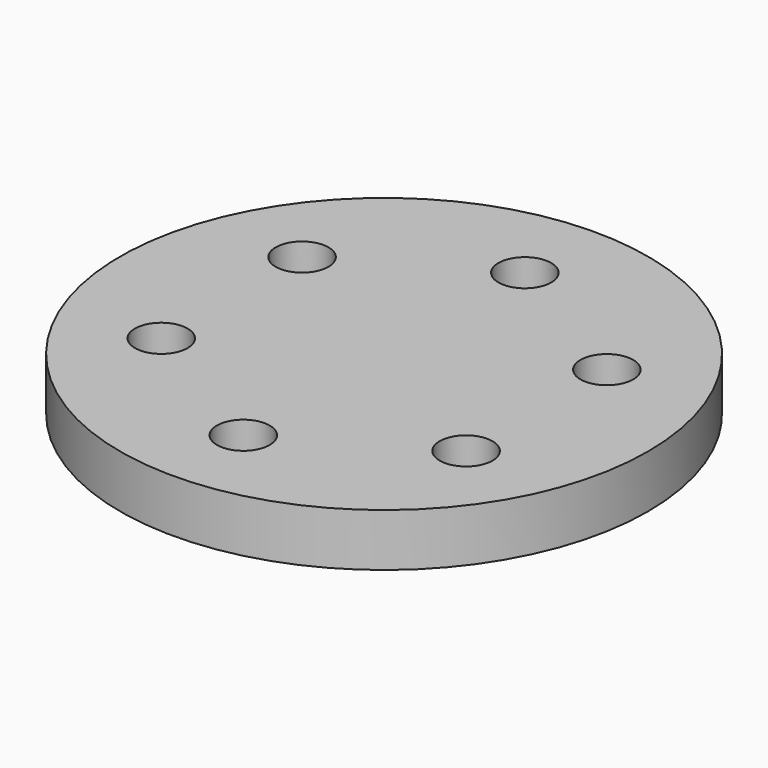
from build123d import *

# Parameters (mm, degrees)
F0_R            = 60
F1_DEPTH        = 12
F2_R            = 6
F3_DEPTH        = 12.001
F3_COPIES_COUNT = 6


# Not quite as in the source:
# - a pattern or mirror of a feature is missing from the dataset's text; its kind, count and spacing are read off the source's solid


with BuildPart() as f1:
    # F0 (on Top) → F1 (new body)
    with BuildSketch(Plane.XY):
        Circle(F0_R)
    extrude(amount=F1_DEPTH)

    # F2 (on face) → F3 (cut, through all)
    with BuildSketch(Plane.XY.offset(12)):
        with Locations((0, 40)):
            Circle(F2_R)
    f3 = extrude(amount=-F3_DEPTH, mode=Mode.SUBTRACT)

    # F3_copies: F3 ×6 about axis
    f3_copies_axis = Axis((0, 0, 0), (0, 0, 1))
    for i in range(1, F3_COPIES_COUNT):
        add(f3.rotate(f3_copies_axis, i * 360 / F3_COPIES_COUNT), mode=Mode.SUBTRACT)


solid = f1.part
